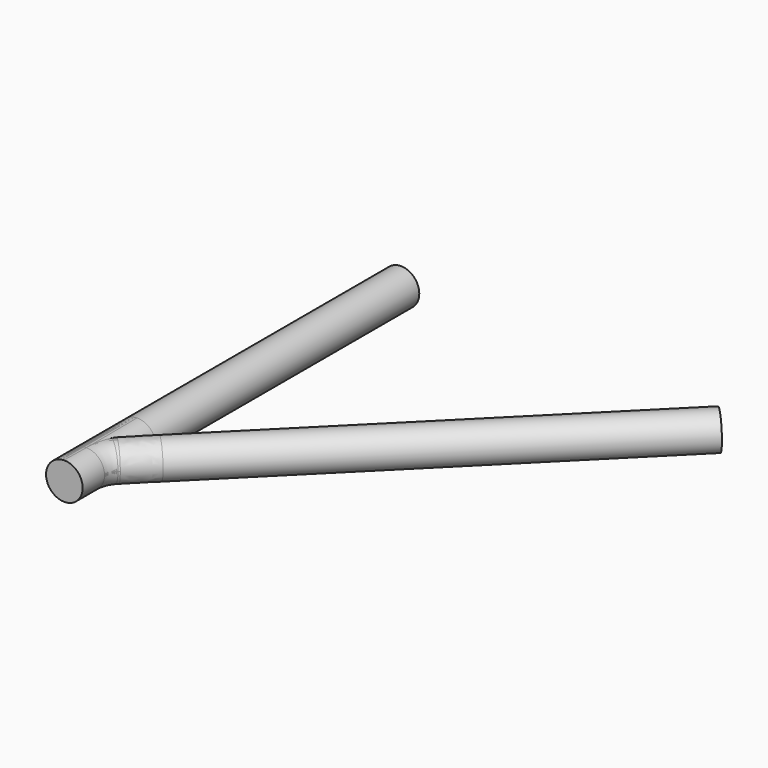
from build123d import *
from build123d import SkipClean  # not in build123d's __all__

# Parameters (mm, degrees)
F1_R     = 50.8
F5_DEPTH = 1219.2
F6_DEPTH = 914.4


with BuildPart() as f2:
    # F2: sweep along a path in F0
    with BuildLine(Plane.XY) as f2_path:
        Line((0, 0), (0, 76.2))
        ThreePointArc((0, 76.2), (7.733839, 115.080638), (29.757951, 148.042052))
        Line((29.757951, 148.042052), (95.701279, 213.98538))
    # F1 (on Front) → F2 (sweep)
    with BuildSketch(Plane.XZ):
        Circle(F1_R)
    sweep(path=f2_path.line)

    # F3: sweep along a path in F0
    with BuildLine(Plane.XY) as f3_path:
        Line((0, 0), (0, 76.2))
        Line((0, 76.2), (0, 254))
    # F1 (on Front) → F3 (sweep)
    with BuildSketch(Plane.XZ):
        Circle(F1_R)
    with SkipClean():  # cleaning this boolean's faces spoils the solid; the shape is the same uncleaned
        sweep(path=f3_path.line)


with BuildPart() as f4_1:
    # F4: copy of F2
    add(f2.part, clean=False)

    # F5 (add): a face of the model
    f5_faces = [f2.part.faces().sort_by_distance(p)[0] for p in [
        (95.701279, 213.98538, 0),
    ]]
    extrude(f5_faces, amount=F5_DEPTH)

    # F6 (add): a face of the model
    f6_faces = [f2.part.faces().sort_by_distance(p)[0] for p in [
        (0, 254, 0),
    ]]
    extrude(f6_faces, amount=F6_DEPTH)


solid = Compound([f2.part, f4_1.part])
